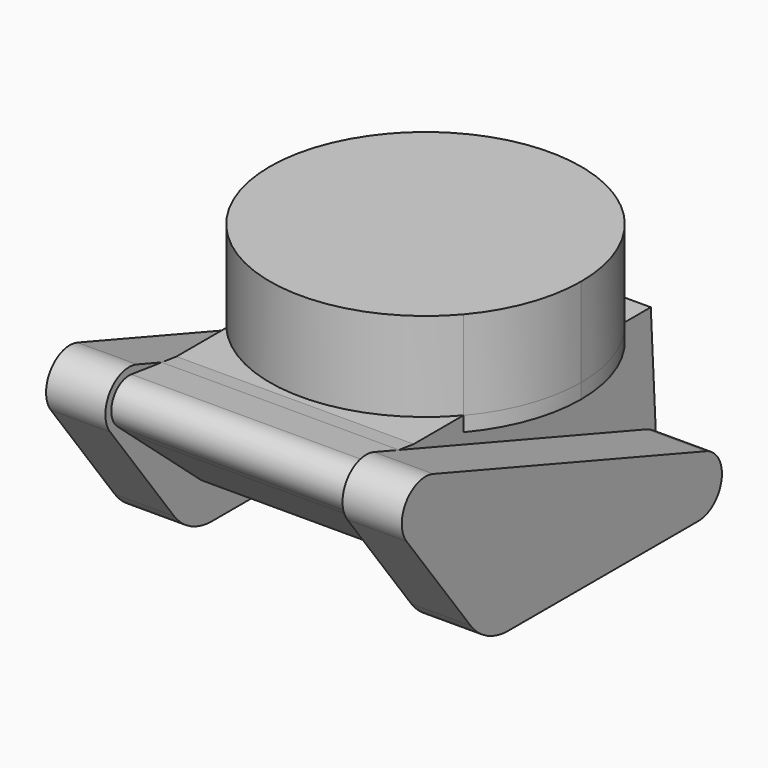
from build123d import *

# Parameters (mm, degrees)
F1_DEPTH      = 40
F2_START      = 40
F2_DEPTH      = 20
F6_DEPTH      = 5
F7_DEPTH      = 30
F7_DEPTH_BACK = 5


with BuildPart() as f1:
    # F0 (on Right) → F1 (new body)
    with BuildSketch(Plane.YZ):
        with BuildLine():
            ThreePointArc((-67.5, 40), (-69.3699394637, 44.9550396928), (-74.047311562, 47.4392462481))
            ThreePointArc((-74.047311562, 47.4392462481), (-81.8542766067, 43.0444855394), (-79.8809353009, 34.3055754823))
            ThreePointArc((-79.8809353009, 34.3055754823), (-71.8660739285, 33.1861532613), (-67.5, 40))
        make_face()
        with BuildLine():
            Line((-22.5329362893, 0.2582503971), (32.5064382574, -6.6216714212))
            ThreePointArc((32.5064382574, -6.6216714212), (31.6956764696, 5.5711947285), (43.2852062494, 9.4449679671))
            Line((43.2852062494, 9.4449679671), (-61.2288449484, 45.7976814272))
            Line((-61.2288449484, 45.7976814272), (-67.4865130573, 46.5990540202))
            ThreePointArc((-67.4865130573, 46.5990540202), (-65.6422526902, 43.5259843004), (-65, 40))
            ThreePointArc((-65, 40), (-67.8792292984, 32.9789869239), (-74.8589249231, 30.0009951584))
            Line((-74.8589249231, 30.0009951584), (-58.9579294654, 16.3715704804))
            ThreePointArc((-58.9579294654, 16.3715704804), (-36.7718882692, 29.7377631624), (-20, 10))
            ThreePointArc((-20, 10), (-20.6435892504, 4.9671714819), (-22.5329362893, 0.2582503971))
        make_face()
        with BuildLine():
            ThreePointArc((-65, 40), (-65.6422526902, 43.5259843004), (-67.4865130573, 46.5990540202))
            Line((-67.4865130573, 46.5990540202), (-74.047311562, 47.4392462481))
            ThreePointArc((-74.047311562, 47.4392462481), (-69.3699394637, 44.9550396928), (-67.5, 40))
            ThreePointArc((-67.5, 40), (-71.8660739285, 33.1861532613), (-79.8809353009, 34.3055754823))
            Line((-79.8809353009, 34.3055754823), (-74.8589249231, 30.0009951584))
            ThreePointArc((-74.8589249231, 30.0009951584), (-67.8792292984, 32.9789869239), (-65, 40))
        make_face()
        with BuildLine():
            Line((-40.9302605094, 2.5579159246), (-22.5329362893, 0.2582503971))
            ThreePointArc((-22.5329362893, 0.2582503971), (-20.6435892504, 4.9671714819), (-20, 10))
            ThreePointArc((-20, 10), (-36.7718882692, 29.7377631624), (-58.9579294654, 16.3715704804))
            Line((-58.9579294654, 16.3715704804), (-44.8809353009, 4.3055754823))
            ThreePointArc((-44.8809353009, 4.3055754823), (-43.1339260715, 16.8138467387), (-32.5, 10))
            ThreePointArc((-32.5, 10), (-35.0364807757, 4.3774136814), (-40.9302605094, 2.5579159246))
        make_face()
        with BuildLine():
            ThreePointArc((-44.8809353009, 4.3055754823), (-43.0341518863, 3.1411427824), (-40.9302605094, 2.5579159246))
            ThreePointArc((-40.9302605094, 2.5579159246), (-35.0364807757, 4.3774136814), (-32.5, 10))
            ThreePointArc((-32.5, 10), (-43.1339260715, 16.8138467387), (-44.8809353009, 4.3055754823))
        make_face()
        with BuildLine():
            ThreePointArc((47.4883448123, 0.4179616875), (34.8816802289, 5.4820436628), (39.0697394906, -7.4420840754))
            ThreePointArc((39.0697394906, -7.4420840754), (44.9635192243, -5.6225863186), (47.5, 0))
            ThreePointArc((47.5, 0), (47.4970856368, 0.2090620815), (47.4883448123, 0.4179616875))
        make_face()
        with BuildLine():
            ThreePointArc((43.2852062494, 9.4449679671), (31.6956764696, 5.5711947285), (32.5064382574, -6.6216714212))
            Line((32.5064382574, -6.6216714212), (39.0697394906, -7.4420840754))
            ThreePointArc((39.0697394906, -7.4420840754), (34.8816802289, 5.4820436628), (47.4883448123, 0.4179616875))
            Line((47.4883448123, 0.4179616875), (47.1197372514, 7.0220610558))
            ThreePointArc((47.1197372514, 7.0220610558), (45.3416600218, 8.4537960829), (43.2852062494, 9.4449679671))
        make_face()
        with BuildLine():
            ThreePointArc((43.2852062494, 9.4449679671), (45.3416600218, 8.4537960829), (47.1197372514, 7.0220610558))
            Line((47.1197372514, 7.0220610558), (45, 45))
            Line((45, 45), (-55, 45))
            Line((-55, 45), (-61.2288449484, 45.7976814272))
            Line((-61.2288449484, 45.7976814272), (43.2852062494, 9.4449679671))
        make_face()
    extrude(amount=F1_DEPTH)

    # F4: F1 across plane


with BuildPart() as f2:
    # F0 (on Right) → F2 (new body)
    with BuildSketch(Plane.YZ.offset(F2_START)):
        with BuildLine():
            ThreePointArc((-71.7147937506, 49.4449679671), (-83.0742850398, 45.8996543201), (-83, 34))
            ThreePointArc((-83, 34), (-79.4089324294, 31.0244044859), (-74.8589249231, 30.0009951584))
            Line((-74.8589249231, 30.0009951584), (-79.8809353009, 34.3055754823))
            ThreePointArc((-79.8809353009, 34.3055754823), (-81.8542766067, 43.0444855394), (-74.047311562, 47.4392462481))
            Line((-74.047311562, 47.4392462481), (-67.4865130573, 46.5990540202))
            ThreePointArc((-67.4865130573, 46.5990540202), (-69.4162960131, 48.2959176579), (-71.7147937506, 49.4449679671))
        make_face()
        with BuildLine():
            Line((-67.4865130573, 46.5990540202), (-61.2288449484, 45.7976814272))
            Line((-61.2288449484, 45.7976814272), (-71.7147937506, 49.4449679671))
            ThreePointArc((-71.7147937506, 49.4449679671), (-69.4162960131, 48.2959176579), (-67.4865130573, 46.5990540202))
        make_face()
        with BuildLine():
            Line((-83, 34), (-56, -2))
            ThreePointArc((-56, -2), (-59.7457048141, 6.8208269322), (-58.9579294654, 16.3715704804))
            Line((-58.9579294654, 16.3715704804), (-74.8589249231, 30.0009951584))
            ThreePointArc((-74.8589249231, 30.0009951584), (-79.4089324294, 31.0244044859), (-83, 34))
        make_face()
        with BuildLine():
            ThreePointArc((-67.5, 40), (-69.3699394637, 44.9550396928), (-74.047311562, 47.4392462481))
            ThreePointArc((-74.047311562, 47.4392462481), (-81.8542766067, 43.0444855394), (-79.8809353009, 34.3055754823))
            ThreePointArc((-79.8809353009, 34.3055754823), (-71.8660739285, 33.1861532613), (-67.5, 40))
        make_face()
        with BuildLine():
            ThreePointArc((-65, 40), (-65.6422526902, 43.5259843004), (-67.4865130573, 46.5990540202))
            Line((-67.4865130573, 46.5990540202), (-74.047311562, 47.4392462481))
            ThreePointArc((-74.047311562, 47.4392462481), (-69.3699394637, 44.9550396928), (-67.5, 40))
            ThreePointArc((-67.5, 40), (-71.8660739285, 33.1861532613), (-79.8809353009, 34.3055754823))
            Line((-79.8809353009, 34.3055754823), (-74.8589249231, 30.0009951584))
            ThreePointArc((-74.8589249231, 30.0009951584), (-67.8792292984, 32.9789869239), (-65, 40))
        make_face()
        with BuildLine():
            Line((-22.5329362893, 0.2582503971), (32.5064382574, -6.6216714212))
            ThreePointArc((32.5064382574, -6.6216714212), (31.6956764696, 5.5711947285), (43.2852062494, 9.4449679671))
            Line((43.2852062494, 9.4449679671), (-61.2288449484, 45.7976814272))
            Line((-61.2288449484, 45.7976814272), (-67.4865130573, 46.5990540202))
            ThreePointArc((-67.4865130573, 46.5990540202), (-65.6422526902, 43.5259843004), (-65, 40))
            ThreePointArc((-65, 40), (-67.8792292984, 32.9789869239), (-74.8589249231, 30.0009951584))
            Line((-74.8589249231, 30.0009951584), (-58.9579294654, 16.3715704804))
            ThreePointArc((-58.9579294654, 16.3715704804), (-36.7718882692, 29.7377631624), (-20, 10))
            ThreePointArc((-20, 10), (-20.6435892504, 4.9671714819), (-22.5329362893, 0.2582503971))
        make_face()
        with BuildLine():
            ThreePointArc((-44.8809353009, 4.3055754823), (-43.0341518863, 3.1411427824), (-40.9302605094, 2.5579159246))
            ThreePointArc((-40.9302605094, 2.5579159246), (-35.0364807757, 4.3774136814), (-32.5, 10))
            ThreePointArc((-32.5, 10), (-43.1339260715, 16.8138467387), (-44.8809353009, 4.3055754823))
        make_face()
        with BuildLine():
            ThreePointArc((-56, -2), (-48.94427191, -7.88854382), (-40, -10))
            ThreePointArc((-40, -10), (-29.8716978732, -7.2457964742), (-22.5329362893, 0.2582503971))
            Line((-22.5329362893, 0.2582503971), (-40.9302605094, 2.5579159246))
            ThreePointArc((-40.9302605094, 2.5579159246), (-43.0341518863, 3.1411427824), (-44.8809353009, 4.3055754823))
            Line((-44.8809353009, 4.3055754823), (-58.9579294654, 16.3715704804))
            ThreePointArc((-58.9579294654, 16.3715704804), (-59.7457048141, 6.8208269322), (-56, -2))
        make_face()
        with BuildLine():
            ThreePointArc((43.2852062494, 9.4449679671), (31.6956764696, 5.5711947285), (32.5064382574, -6.6216714212))
            Line((32.5064382574, -6.6216714212), (39.0697394906, -7.4420840754))
            ThreePointArc((39.0697394906, -7.4420840754), (34.8816802289, 5.4820436628), (47.4883448123, 0.4179616875))
            Line((47.4883448123, 0.4179616875), (47.1197372514, 7.0220610558))
            ThreePointArc((47.1197372514, 7.0220610558), (45.3416600218, 8.4537960829), (43.2852062494, 9.4449679671))
        make_face()
        with BuildLine():
            ThreePointArc((47.4883448123, 0.4179616875), (34.8816802289, 5.4820436628), (39.0697394906, -7.4420840754))
            ThreePointArc((39.0697394906, -7.4420840754), (44.9635192243, -5.6225863186), (47.5, 0))
            ThreePointArc((47.5, 0), (47.4970856368, 0.2090620815), (47.4883448123, 0.4179616875))
        make_face()
        with BuildLine():
            ThreePointArc((32.5064382574, -6.6216714212), (35.8900556094, -9.1163785083), (40, -10))
            ThreePointArc((40, -10), (47.0710678119, -7.0710678119), (50, 0))
            ThreePointArc((50, 0), (49.2519558071, 3.7949062891), (47.1197372514, 7.0220610558))
            Line((47.1197372514, 7.0220610558), (47.4883448123, 0.4179616875))
            ThreePointArc((47.4883448123, 0.4179616875), (47.4970856368, 0.2090620815), (47.5, 0))
            ThreePointArc((47.5, 0), (44.9635192243, -5.6225863186), (39.0697394906, -7.4420840754))
            Line((39.0697394906, -7.4420840754), (32.5064382574, -6.6216714212))
        make_face()
        with BuildLine():
            Line((-40, -10), (40, -10))
            ThreePointArc((40, -10), (35.8900556094, -9.1163785083), (32.5064382574, -6.6216714212))
            Line((32.5064382574, -6.6216714212), (-22.5329362893, 0.2582503971))
            ThreePointArc((-22.5329362893, 0.2582503971), (-29.8716978732, -7.2457964742), (-40, -10))
        make_face()
        with BuildLine():
            Line((-40.9302605094, 2.5579159246), (-22.5329362893, 0.2582503971))
            ThreePointArc((-22.5329362893, 0.2582503971), (-20.6435892504, 4.9671714819), (-20, 10))
            ThreePointArc((-20, 10), (-36.7718882692, 29.7377631624), (-58.9579294654, 16.3715704804))
            Line((-58.9579294654, 16.3715704804), (-44.8809353009, 4.3055754823))
            ThreePointArc((-44.8809353009, 4.3055754823), (-43.1339260715, 16.8138467387), (-32.5, 10))
            ThreePointArc((-32.5, 10), (-35.0364807757, 4.3774136814), (-40.9302605094, 2.5579159246))
        make_face()
    extrude(amount=F2_DEPTH)


with BuildPart() as f3_1:
    # F3: instance of F2
    add(f2.part.mirror(Plane.YZ))


with BuildPart() as f1_1:
    add(f1.part)
    add(f1.part.mirror(Plane.YZ))

    # F5 (on face) → F6 (cut)
    with BuildSketch(Plane.XY.offset(45)):
        with BuildLine():
            Line((40, -34.0036762718), (40, 34.0036762718))
            ThreePointArc((40, 34.0036762718), (33.9687352606, 40.0296768011), (27.041634566, 45))
            Line((27.041634566, 45), (-27.041634566, 45))
            ThreePointArc((-27.041634566, 45), (-33.9687352606, 40.0296768011), (-40, 34.0036762718))
            Line((-40, 34.0036762718), (-40, -34.0036762718))
            ThreePointArc((-40, -34.0036762718), (0, -52.5), (40, -34.0036762718))
        make_face()
        with BuildLine():
            Line((-27.041634566, 45), (27.041634566, 45))
            ThreePointArc((27.041634566, 45), (0, 52.5), (-27.041634566, 45))
        make_face()
    extrude(amount=-F6_DEPTH, mode=Mode.SUBTRACT)


with BuildPart() as f7:
    # F5 (on face) → F7 (new body, two sides)
    with BuildSketch(Plane.XY.offset(45)) as f7_sk:
        with BuildLine():
            ThreePointArc((40, -34.0036762718), (49.2760083611, -18.1142209327), (52.5, 0))
            ThreePointArc((52.5, 0), (49.2760083611, 18.1142209327), (40, 34.0036762718))
            Line((40, 34.0036762718), (40, -34.0036762718))
        make_face()
        with BuildLine():
            Line((40, -34.0036762718), (40, 34.0036762718))
            ThreePointArc((40, 34.0036762718), (33.9687352606, 40.0296768011), (27.041634566, 45))
            Line((27.041634566, 45), (-27.041634566, 45))
            ThreePointArc((-27.041634566, 45), (-33.9687352606, 40.0296768011), (-40, 34.0036762718))
            Line((-40, 34.0036762718), (-40, -34.0036762718))
            ThreePointArc((-40, -34.0036762718), (0, -52.5), (40, -34.0036762718))
        make_face()
        with BuildLine():
            Line((-27.041634566, 45), (27.041634566, 45))
            ThreePointArc((27.041634566, 45), (0, 52.5), (-27.041634566, 45))
        make_face()
        with BuildLine():
            ThreePointArc((-40, 34.0036762718), (-52.5, 0), (-40, -34.0036762718))
            Line((-40, -34.0036762718), (-40, 34.0036762718))
        make_face()
    extrude(amount=F7_DEPTH)
    extrude(f7_sk.sketch, amount=-F7_DEPTH_BACK)


solid = Compound([f2.part, f3_1.part, f1_1.part, f7.part])
